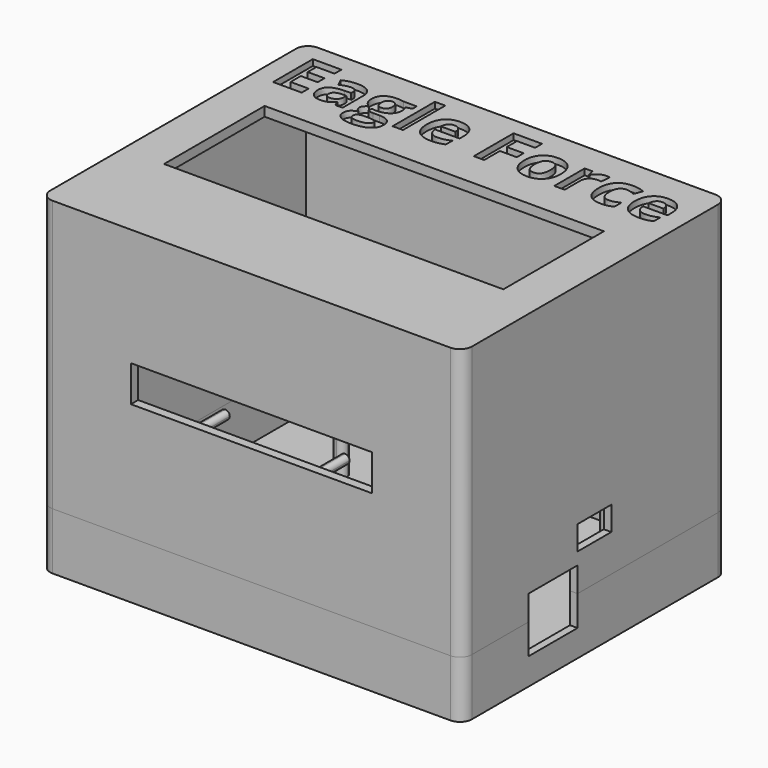
from build123d import *

# Parameters (mm, degrees)
F0_W          = 88.9
F0_H          = 69.85
F1_DEPTH      = 10
F1_DEPTH_BACK = 2
F2_W          = 85.725
F2_H          = 66.04
F3_DEPTH      = 8.89
F4_R          = 2.54
F7_DEPTH      = 9.9568
F8_DEPTH      = 15.24
F10_W         = 88.8999849558
F10_H         = 69.8501616716
F11_DEPTH     = 57.15
F13_W         = 12.9504366778
F13_H         = 5.2537366375
F14_DEPTH     = 3.0226
F15_W         = 85.725069046
F15_H         = 66.0407468677
F16_DEPTH     = 55.88
F17_R         = 2.54
F19_DEPTH     = 6.1722
F21_W         = 8.89
F21_H         = 5.08
F22_DEPTH     = 7.62
F24_DEPTH     = 5.08
F25_TEXT_SIZE = 14.663917116
F26_DEPTH     = 1.27
F27_DEPTH     = 8.89
F28_DEPTH     = 6.096
F29_DEPTH     = 10.16
F9_W          = 12.9504366778
F9_H          = 6.3706803974
F9_H_2        = 5.2401281521
F30_DEPTH     = 6.858


# Not quite as in the source:
# - Text() gives the source's letters only with a copy of the font that has no kerning and outlines rounded to 1/6400 em; it was checked with that copy


with BuildPart() as f1:
    # F0 (on Top) → F1 (new body, two sides)
    with BuildSketch(Plane.XY) as f1_sk:
        Rectangle(F0_W, F0_H)
    extrude(amount=F1_DEPTH)
    extrude(f1_sk.sketch, amount=-F1_DEPTH_BACK)

    # F2 (on face) → F3 (cut)
    with BuildSketch(Plane.XY.offset(10)):
        Rectangle(F2_W, F2_H)
    extrude(amount=-F3_DEPTH, mode=Mode.SUBTRACT)

    # F4
    f4_edges = [f1.edges().sort_by_distance(p)[0] for p in [
        (44.45, 34.925, 4),
        (44.45, -34.925, 4),
        (-44.45, -34.925, 4),
        (-44.45, 34.925, 4),
    ]]
    fillet(f4_edges, radius=F4_R)

    # F2 (on face) → F7 (cut)
    with BuildSketch(Plane.XY.offset(10)):
        Rectangle(F2_W, F2_H)
    extrude(amount=-F7_DEPTH, mode=Mode.SUBTRACT)

    # F6 (on face) → F8 (join)
    with BuildSketch(Plane.XY):
        with BuildLine():
            ThreePointArc((28.9179, 24.384), (28.5459256121, 25.2820256121), (27.6479, 25.654))
            Line((27.6479, 25.654), (27.6479, 24.384))
            Line((27.6479, 24.384), (26.3779, 24.384))
            ThreePointArc((26.3779, 24.384), (27.6479, 23.114), (28.9179, 24.384))
        make_face()
        with BuildLine():
            ThreePointArc((-23.1521, 19.304), (-25.3201256121, 20.2020256121), (-24.4221, 18.034))
            ThreePointArc((-24.4221, 18.034), (-23.5240743879, 18.4059743879), (-23.1521, 19.304))
        make_face()
        with BuildLine():
            ThreePointArc((-24.4221, -7.366), (-25.6921, -8.636), (-24.4221, -9.906))
            Line((-24.4221, -9.906), (-24.4221, -8.636))
            Line((-24.4221, -8.636), (-24.4221, -7.366))
        make_face()
        with BuildLine():
            Line((-24.4221, -8.636), (-24.4221, -9.906))
            ThreePointArc((-24.4221, -9.906), (-23.5240743879, -9.5340256121), (-23.1521, -8.636))
            ThreePointArc((-23.1521, -8.636), (-23.5240743879, -7.7379743879), (-24.4221, -7.366))
            Line((-24.4221, -7.366), (-24.4221, -8.636))
        make_face()
        with BuildLine():
            ThreePointArc((27.6479, -23.876), (27.2759256121, -22.9779743879), (26.3779, -22.606))
            Line((26.3779, -22.606), (26.3779, -23.876))
            Line((26.3779, -23.876), (25.1079, -23.876))
            ThreePointArc((25.1079, -23.876), (26.3779, -25.146), (27.6479, -23.876))
        make_face()
        with BuildLine():
            Line((26.3779, -23.876), (26.3779, -22.606))
            ThreePointArc((26.3779, -22.606), (25.4798743879, -22.9779743879), (25.1079, -23.876))
            Line((25.1079, -23.876), (26.3779, -23.876))
        make_face()
        with BuildLine():
            Line((27.6479, 24.384), (27.6479, 25.654))
            ThreePointArc((27.6479, 25.654), (26.7498743879, 25.2820256121), (26.3779, 24.384))
            Line((26.3779, 24.384), (27.6479, 24.384))
        make_face()
    extrude(amount=F8_DEPTH)

    # F9 (on face) → F30 (cut)
    with BuildSketch(Plane.YZ.offset(44.45)):
        with Locations((-11.0509016085, 6.8146598013)):
            Rectangle(F9_W, F9_H)
        with Locations((-11.0509016085, 12.620064076)):
            Rectangle(F9_W, F9_H_2)
    extrude(amount=-F30_DEPTH, mode=Mode.SUBTRACT)


with BuildPart() as f11:
    # F10 (on face) → F11 (new body)
    with BuildSketch(Plane.XY.offset(10)):
        Rectangle(F10_W, F10_H)
    extrude(amount=F11_DEPTH)

    # F13 (on face) → F14 (cut)
    with BuildSketch(Plane.YZ.offset(44.45)):
        with Locations((-11.0509016085, 12.6268683188)):
            Rectangle(F13_W, F13_H)
    extrude(amount=-F14_DEPTH, mode=Mode.SUBTRACT)

    # F15 (on offset) → F16 (cut)
    with BuildSketch(Plane.XY.offset(65.15)):
        Rectangle(F15_W, F15_H)
    extrude(amount=-F16_DEPTH, mode=Mode.SUBTRACT)

    # F17
    f17_edges = [f11.edges().sort_by_distance(p)[0] for p in [
        (44.449992, -34.925081, 38.575),
        (-44.449992, -34.925081, 38.575),
        (-44.449992, 34.925081, 38.575),
        (44.449992, 34.925081, 38.575),
    ]]
    fillet(f17_edges, radius=F17_R)

    # F18 (on face) → F19 (cut)
    with BuildSketch(Plane.XZ.offset(34.9250808358)):
        Polygon((-12.62634, 34.765), (0, 34.765), (12.62634, 34.765), (25.4, 34.765), (25.4, 42.385), (-25.4, 42.385), (-25.4, 34.765), align=None)
    extrude(amount=-F19_DEPTH, mode=Mode.SUBTRACT)

    # F21 (on face) → F22 (cut)
    with BuildSketch(Plane.YZ.offset(44.4499924779)):
        with Locations((-0.1306832696, 20.3559232764)):
            Rectangle(F21_W, F21_H)
    extrude(amount=-F22_DEPTH, mode=Mode.SUBTRACT)

    # F23 (on face) → F24 (cut)
    with BuildSketch(Plane.XY.offset(67.15)):
        Polygon((-35.7500047, -13.2499989), (0, -13.2499989), (35.7500047, -13.2499989), (35.7500047, 13.2499989), (-35.7500047, 13.2499989), align=None)
    extrude(amount=-F24_DEPTH, mode=Mode.SUBTRACT)

    # F25 (on face) → F26 (cut)
    with BuildSketch(Plane.XY.offset(67.15)):
        with Locations((-41.2988741882, 20.7577981055)):
            Text('Eagle Force', F25_TEXT_SIZE, font='Open Sans', font_style=FontStyle.BOLD, text_align=(TextAlign.LEFT, TextAlign.BOTTOM))
    extrude(amount=-F26_DEPTH, mode=Mode.SUBTRACT)

    # F18 (on face) → F27 (join)
    with BuildSketch(Plane.XZ.offset(34.9250808358)):
        with BuildLine():
            ThreePointArc((-11.67384, 33.368), (-11.9528207909, 34.0415192091), (-12.62634, 34.3205))
            ThreePointArc((-12.62634, 34.3205), (-13.2998592091, 32.6944807909), (-11.67384, 33.368))
        make_face()
        with BuildLine():
            ThreePointArc((13.57884, 33.368), (13.2998592091, 34.0415192091), (12.62634, 34.3205))
            ThreePointArc((12.62634, 34.3205), (11.9528207909, 32.6944807909), (13.57884, 33.368))
        make_face()
    extrude(amount=-F27_DEPTH)

    # F20 (on face) → F28 (cut)
    with BuildSketch(Plane(origin=(0, 34.9250808358, 0), x_dir=(-1, 0, 0), z_dir=(0, 1, 0))):
        with BuildLine():
            ThreePointArc((0.6358234934, 24.2496207356), (5.0082821399, 19.8771620892), (9.3807407864, 24.2496207356))
            ThreePointArc((9.3807407864, 24.2496207356), (5.0082821399, 28.6220793821), (0.6358234934, 24.2496207356))
        make_face()
    extrude(amount=-F28_DEPTH, mode=Mode.SUBTRACT)

    # F23 (on face) → F29 (join)
    with BuildSketch(Plane.XY.offset(67.15)):
        with BuildLine():
            ThreePointArc((-37.500052, -14.229969), (-38.3980776121, -16.3979946121), (-36.230052, -15.499969))
            Line((-36.230052, -15.499969), (-37.500052, -15.499969))
            Line((-37.500052, -15.499969), (-37.500052, -14.229969))
        make_face()
        with BuildLine():
            Line((-37.500052, -15.499969), (-36.230052, -15.499969))
            ThreePointArc((-36.230052, -15.499969), (-36.6020263879, -14.6019433879), (-37.500052, -14.229969))
            Line((-37.500052, -14.229969), (-37.500052, -15.499969))
        make_face()
        with BuildLine():
            Line((37.500052, 15.499969), (37.500052, 14.229969))
            ThreePointArc((37.500052, 14.229969), (38.3980776121, 14.6019433879), (38.770052, 15.499969))
            ThreePointArc((38.770052, 15.499969), (37.500052, 16.769969), (36.230052, 15.499969))
            Line((36.230052, 15.499969), (37.500052, 15.499969))
        make_face()
        with BuildLine():
            ThreePointArc((36.230052, 15.499969), (36.6020263879, 14.6019433879), (37.500052, 14.229969))
            Line((37.500052, 14.229969), (37.500052, 15.499969))
            Line((37.500052, 15.499969), (36.230052, 15.499969))
        make_face()
    extrude(amount=-F29_DEPTH)


solid = Compound([f1.part, f11.part])
